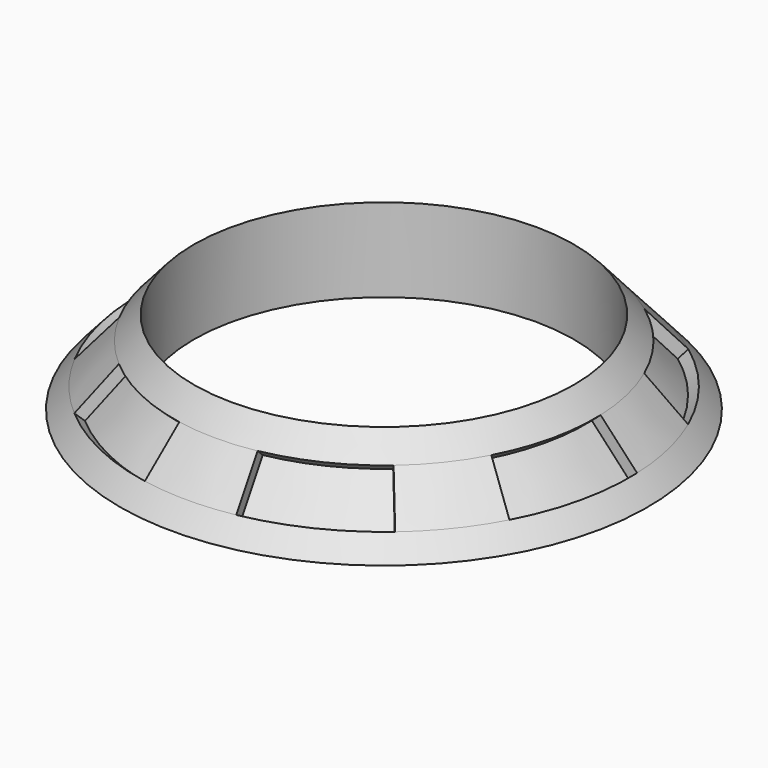
from build123d import *

# Parameters (mm, degrees)
F2_ANGLE_BACK   = 15
F2_ANGLE        = 30
F2_COPIES_COUNT = 7


# Not quite as in the source:
# - a pattern or mirror of a feature is missing from the dataset's text; its kind, count and spacing are read off the source's solid


with BuildPart() as f1:
    # F0 (on Right) → F1 (revolve)
    with BuildSketch(Plane.YZ):
        Polygon((9.3, 4.0896662887), (9.3, 0), (12.9161745474, 0), (12.0366714414, 0.9946627731), (11.620462189, 0.6266412283), (9.8856947209, 2.5885542775), (10.3019039734, 2.9565758223), align=None)
        Polygon((11.620462189, 0.6266412283), (12.0366714414, 0.9946627731), (10.3019039734, 2.9565758223), (9.8856947209, 2.5885542775), align=None)
    revolve(axis=Axis((0, 0, 2.1812447902), (0, 0, 1)))

    # F0 (on Right) → F2 (revolve, cut)
    with BuildSketch(Plane.YZ, mode=Mode.PRIVATE) as f2_sk:
        Polygon((11.620462189, 0.6266412283), (12.0366714414, 0.9946627731), (10.3019039734, 2.9565758223), (9.8856947209, 2.5885542775), align=None)
    f2 = revolve(f2_sk.sketch.rotate(Axis((0, 0, 2.1812447902), (0, 0, -1)), -F2_ANGLE_BACK), axis=Axis((0, 0, 2.1812447902), (0, 0, -1)), revolution_arc=F2_ANGLE, mode=Mode.SUBTRACT)

    # F2_copies: F2 ×7 about axis
    f2_copies_axis = Axis((0, 0, 0), (0, 0, 1))
    for i in range(1, F2_COPIES_COUNT):
        add(f2.rotate(f2_copies_axis, i * 360 / F2_COPIES_COUNT), mode=Mode.SUBTRACT)


solid = f1.part
